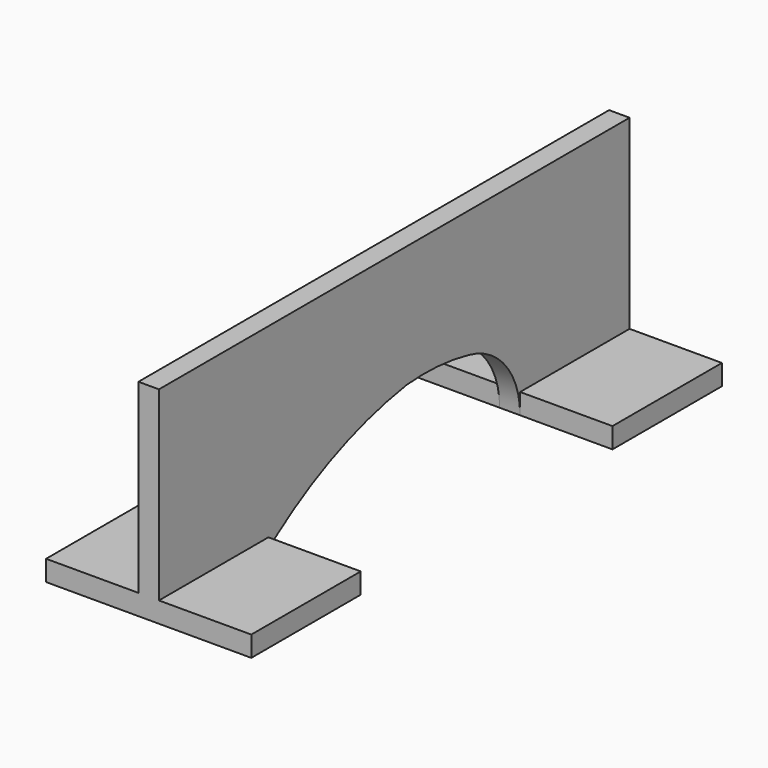
from build123d import *

# Parameters (mm, degrees)
F1_DEPTH = 3
F2_ANGLE = 90
F7_W     = 20
F7_H     = 3
F8_DEPTH = 15


# Not quite as in the source:
# - ends of sketch curves that miss each other by under 0.0002 mm in the source are joined


with BuildPart() as f1:
    # F0 (on Top) → F1 (new body)
    with BuildSketch(Plane.XY):
        with BuildLine():
            ThreePointArc((2.5843454528, -32.7194872419), (1.4841670751, -33.7858704597), (0, -34.1664144431))
            Line((0, -34.1664144431), (0, -54.1664144431))
            Line((0, -54.1664144431), (30.1699284464, -54.1664144431))
            Line((30.1699284464, -54.1664144431), (30.1699284464, 31.83347))
            Line((30.1699284464, 31.83347), (0, 31.83347))
            Line((0, 31.83347), (0, 11.83347))
            ThreePointArc((0, 11.83347), (7.4846118013, 9.165784114), (11.5946270955, 2.3655094074))
            ThreePointArc((11.5946270955, 2.3655094074), (12.4147060347, -3.2443514979), (12.338869311, -8.913329936))
            ThreePointArc((12.338869311, -8.913329936), (8.8720047217, -21.3943156457), (2.5843454528, -32.7194872419))
        make_face()
    extrude(amount=F1_DEPTH)


with BuildPart() as f1_1:
    # F2: moved
    add(f1.part.rotate(Axis((0, -44.1664144431, 3), (0, -1, 0)), F2_ANGLE))

    # F7 (on 3pt) → F8 (join, symmetric)
    with BuildSketch(Plane.YZ.offset(1.5)):
        with Locations((-44.1664144431, 4.5)):
            Rectangle(F7_W, F7_H)
        with Locations((21.83347, 4.5)):
            Rectangle(F7_W, F7_H)
    extrude(amount=F8_DEPTH, both=True)


solid = f1_1.part
